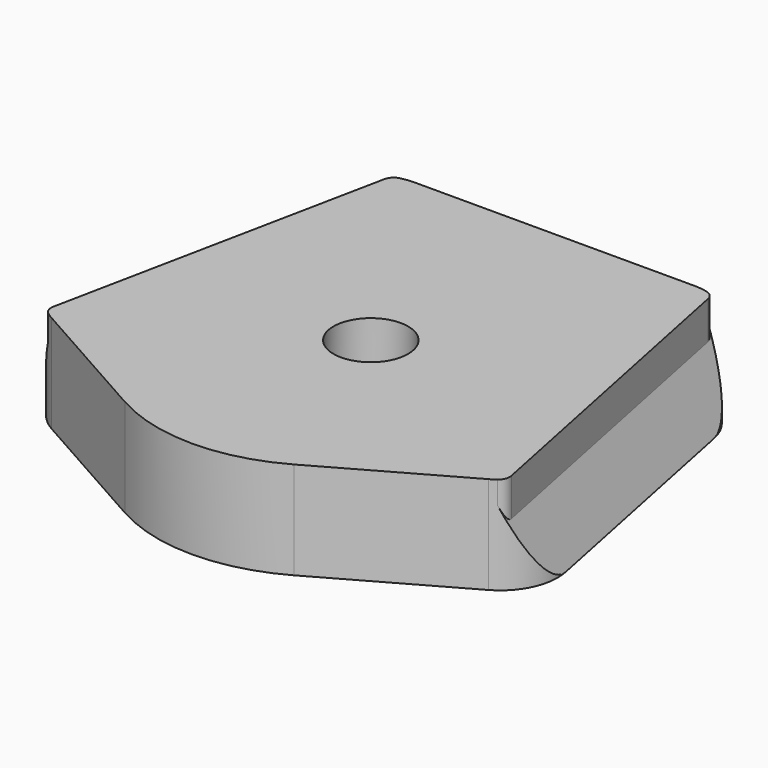
from build123d import *

# Parameters (mm, degrees)
F0_R     = 3.25
F1_DEPTH = 8.5
F2_R     = 6
F2_R_2   = 3.25
F3_DEPTH = 4
F7_DEPTH = 48.701737703
F8_R     = 1


# Not quite as in the source:
# - a pattern or mirror of a feature is missing from the dataset's text; its kind, count and spacing are read off the source's solid


with BuildPart() as f1:
    # F0 (on Top) → F1 (new body)
    with BuildSketch(Plane.XY):
        with BuildLine():
            Line((21.4749827509, -25.6324591351), (17.0744521737, -4.0031603279))
            ThreePointArc((17.0744521737, -4.0031603279), (15.3383552934, -1.1280367796), (12.1748286506, 0))
            Line((12.1748286506, 0), (0, 0))
            Line((0, 0), (-12.1748286506, 0))
            ThreePointArc((-12.1748286506, 0), (-15.3383552934, -1.1280367796), (-17.0744521737, -4.0031603279))
            Line((-17.0744521737, -4.0031603279), (-21.4749827509, -25.6324591351))
            ThreePointArc((-21.4749827509, -25.6324591351), (-21.1230164973, -28.7074742953), (-19.0284610173, -30.9861659857))
            Line((-19.0284610173, -30.9861659857), (-7.3593053684, -37.5563976295))
            ThreePointArc((-7.3593053684, -37.5563976295), (0, -39.4857960942), (7.3593053684, -37.5563976295))
            Line((7.3593053684, -37.5563976295), (19.0284610173, -30.9861659857))
            ThreePointArc((19.0284610173, -30.9861659857), (21.1230164973, -28.7074742953), (21.4749827509, -25.6324591351))
        make_face()
        with Locations((0, -20)):
            Circle(F0_R, mode=Mode.SUBTRACT)
    extrude(amount=F1_DEPTH)

    # F2 (on face) → F3 (cut)
    with BuildSketch(Plane(origin=(0, 0, 0), x_dir=(1, 0, 0), z_dir=(0, 0, -1))):
        with Locations((0, 20)):
            Circle(F2_R)
        with Locations((0, 20)):
            Circle(F2_R_2, mode=Mode.SUBTRACT)
    extrude(amount=-F3_DEPTH, mode=Mode.SUBTRACT)

    # F6 (on face) → F7 (cut, through all)
    with BuildSketch(Plane(origin=(-8.8517973086, -43.5079737791, 0), x_dir=(-0.9799247046, 0.1993679344, 0), z_dir=(0.1993679344, 0.9799247046, 0))):
        Polygon((15.9335756971, 0), (15.9335756971, 8.5), (13.6335756971, 8.5), (13.6335756971, 5.2), align=None)
    f7 = extrude(amount=F7_DEPTH, mode=Mode.SUBTRACT)

    # F7_copies: F7 across plane
    add(f7.mirror(Plane(origin=(0, 0, 0), x_dir=(0, 0, 1), z_dir=(1, 0, 0))), mode=Mode.SUBTRACT)

    # F8
    f8_edges = [f1.edges().sort_by_distance(p)[0] for p in [
        (-20.060161, -30.214847, 6.85),
        (-13.98162, -0.337865, 6.85),
        (20.060161, -30.214847, 6.85),
        (13.98162, -0.337865, 6.85),
    ]]
    fillet(f8_edges, radius=F8_R)


solid = f1.part
